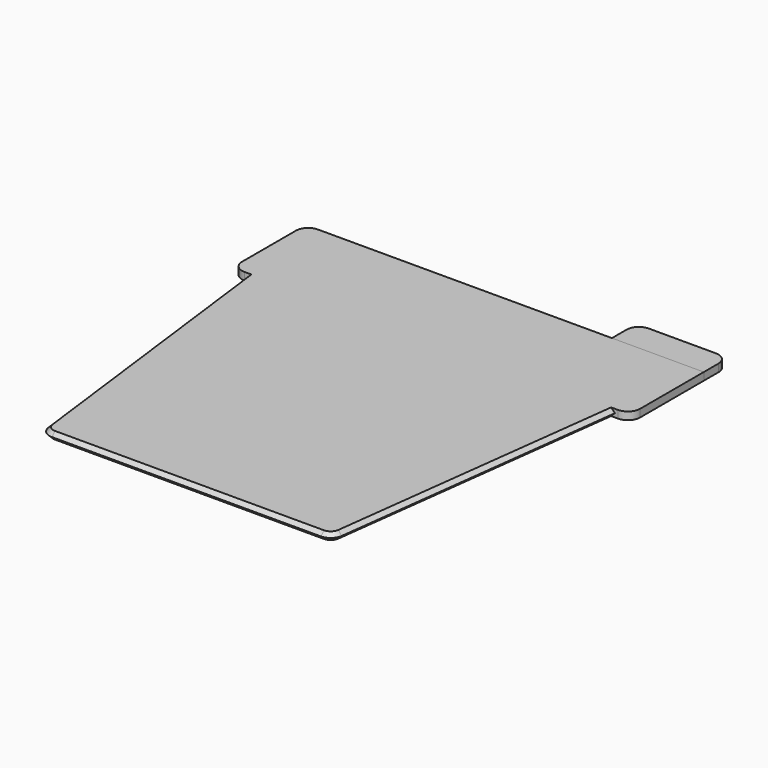
from build123d import *

# Parameters (mm, degrees)
F2_DEPTH = 3.175
F3_W     = 38.1
F3_H     = 12.7
F4_DEPTH = 3.175
F5_R     = 5.08
F5_2_R   = 5.08
F6_SIZE  = 1.58749


# Not quite as in the source:
# - a fillet or chamfer is up to 0.001 mm smaller than in the source, because OpenCascade refuses the exact size


with BuildPart() as f2:
    # F1 (on face) → F2 (new body)
    with BuildSketch(Plane.XY):
        Polygon((82.55, 82.55), (-82.55, 82.55), (-82.55, 44.45), (-76.2, 44.45), (-60.198, -82.55), (60.325, -82.55), (76.2, 44.45), (82.55, 44.45), align=None)
    extrude(amount=F2_DEPTH)

    # F5
    f5_edges = [f2.edges().sort_by_distance(p)[0] for p in [
        (-82.55, 44.45, 1.5875),
        (-82.55, 82.55, 1.5875),
        (82.55, 44.45, 1.5875),
        (60.325, -82.55, 1.5875),
        (-60.198, -82.55, 1.5875),
    ]]
    fillet(f5_edges, radius=F5_R)

    # F6 (size 1.5875 in the source; OpenCascade refuses exactly that, so slightly less here)
    f6_edges = [f2.edges().sort_by_distance(p)[0] for p in [
        (0.061276, -82.55, 0),
        (-55.717914, -82.55, 1.5875),
        (55.840466, -82.55, 1.5875),
        (0.061276, -82.55, 3.175),
        (-59.077996, -81.28002, 0),
        (-60.758063, -78.105059, 1.5875),
        (-59.077996, -81.28002, 3.175),
        (59.202423, -81.278365, 0),
        (60.881238, -78.100096, 1.5875),
        (59.202423, -81.278365, 3.175),
    ]]
    chamfer(f6_edges, length=F6_SIZE)


with BuildPart() as f4:
    # F3 (on face) → F4 (new body)
    with BuildSketch(Plane.XY):
        with Locations((63.5, 88.9)):
            Rectangle(F3_W, F3_H)
    extrude(amount=F4_DEPTH)

    # F5#2
    f5_2_edges = [f4.edges().sort_by_distance(p)[0] for p in [
        (44.45, 95.25, 1.5875),
        (82.55, 95.25, 1.5875),
    ]]
    fillet(f5_2_edges, radius=F5_2_R)


solid = Compound([f2.part, f4.part])
